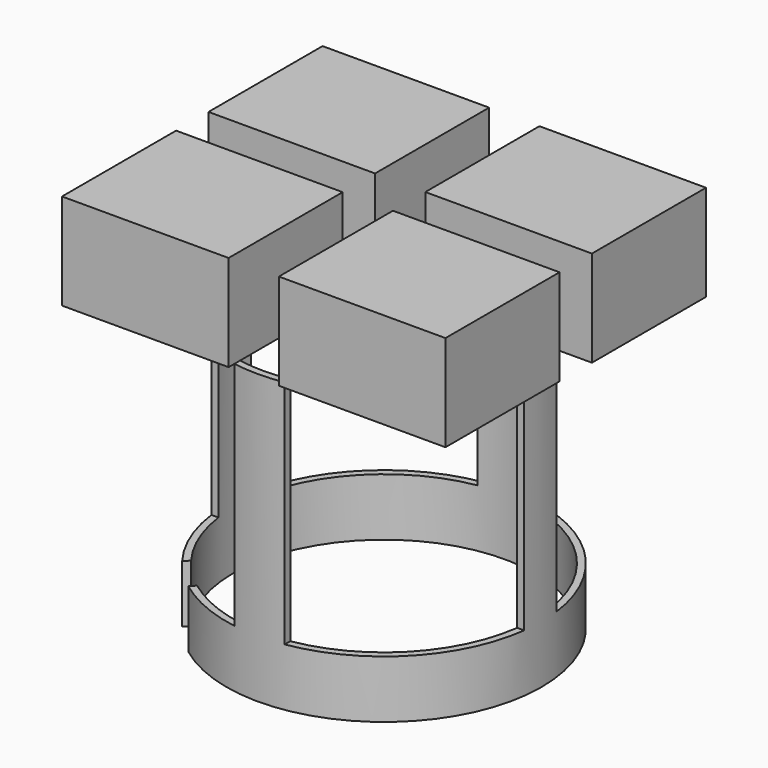
from build123d import *

# Parameters (mm, degrees)
F0_R      = 41
F1_DEPTH  = 75
F2_T      = -1.8
F3_W      = 43.3271373622
F3_H      = 37.0817845687
F4_DEPTH  = 25
F5_FACE_W = 43.3271373622
F5_FACE_H = 37.0817845687
F4_FACE_W = 43.3271373622
F4_FACE_H = 37.0817845687
F6_FACE_W = 43.3271373622
F6_FACE_H = 37.0817845687
F7_DEPTH  = 60
F10_DEPTH = 25


with BuildPart() as f1:
    # F0 (on Top) → F1 (new body)
    with BuildSketch(Plane.XY):
        Circle(F0_R)
    extrude(amount=F1_DEPTH)

    # F2
    f2_openings = [f1.faces().sort_by_distance(p)[0] for p in [
        (0, 0, 75),
        (0, 0, 0),
    ]]
    offset(amount=F2_T, openings=f2_openings)

    # F5_face (on face) + F4_face (on face) + F6_face (on face) → F7 (cut)
    with BuildSketch(Plane(origin=(28.2016734127, 23.8104094751, 75), x_dir=(1, 0, 0), z_dir=(0, 0, -1))):
        Rectangle(F5_FACE_W, F5_FACE_H)
    with BuildSketch(Plane(origin=(-28.2016734127, 23.8104094751, 75), x_dir=(1, 0, 0), z_dir=(0, 0, -1))):
        Rectangle(F4_FACE_W, F4_FACE_H)
    with BuildSketch(Plane(origin=(-28.2016734127, -23.8104094751, 75), x_dir=(1, 0, 0), z_dir=(0, 0, -1))):
        Rectangle(F6_FACE_W, F6_FACE_H)
        with Locations((56.4033468254, 0)):
            Rectangle(F6_FACE_W, F6_FACE_H)
    extrude(amount=F7_DEPTH, mode=Mode.SUBTRACT)

    # F9 (on face) → F10 (cut)
    with BuildSketch(Plane(origin=(0, 0, 0), x_dir=(1, 0, 0), z_dir=(0, 0, -1))):
        with BuildLine():
            Line((-26.0766707361, 33.9554976672), (-29.992537573, 30.0396308303))
            Line((-29.992537573, 30.0396308303), (-27.9037735724, 30.0396308303))
            ThreePointArc((-27.9037735724, 30.0396308303), (-26.3760293541, 31.3895695337), (-24.7830693928, 32.6618963239))
            Line((-24.7830693928, 32.6618963239), (-26.0766707361, 33.9554976672))
        make_face()
        with BuildLine():
            ThreePointArc((-24.7830693928, 32.6618963239), (-26.3760293541, 31.3895695337), (-27.9037735724, 30.0396308303))
            Line((-27.9037735724, 30.0396308303), (-25.184530561, 30.0396308303))
            ThreePointArc((-25.184530561, 30.0396308303), (-24.3503464301, 30.7197107528), (-23.497806174, 31.3766331051))
            Line((-23.497806174, 31.3766331051), (-24.7830693928, 32.6618963239))
        make_face()
        with BuildLine():
            Line((-25.184530561, 30.0396308303), (-27.9037735724, 30.0396308303))
            ThreePointArc((-27.9037735724, 30.0396308303), (-28.9669254959, 29.0158099545), (-29.992537573, 27.9543858801))
            Line((-29.992537573, 27.9543858801), (-29.992537573, 25.2405960693))
            ThreePointArc((-29.992537573, 25.2405960693), (-27.6926866813, 27.7444607872), (-25.184530561, 30.0396308303))
        make_face()
        with BuildLine():
            Line((-29.992537573, 25.2405960693), (-29.992537573, 27.9543858801))
            ThreePointArc((-29.992537573, 27.9543858801), (-31.3456683019, 26.4281872005), (-32.6212227873, 24.8365823708))
            Line((-32.6212227873, 24.8365823708), (-31.3362602205, 23.551619804))
            ThreePointArc((-31.3362602205, 23.551619804), (-30.6760251647, 24.4053576105), (-29.992537573, 25.2405960693))
        make_face()
    extrude(amount=-F10_DEPTH, mode=Mode.SUBTRACT)


with BuildPart() as f4:
    # F3 (on face) → F4 (new body)
    with BuildSketch(Plane.XY.offset(75)):
        with Locations((-28.2016734127, 23.8104094751)):
            Rectangle(F3_W, F3_H)
    extrude(amount=F4_DEPTH)


with BuildPart() as f5_1:
    # F5: instance of F4
    add(f4.part.mirror(Plane.YZ))


with BuildPart() as f6_1:
    # F6: instance of F4
    add(f4.part.mirror(Plane.XZ))


with BuildPart() as f6_2:
    # F6: instance of F5_1
    add(f5_1.part.mirror(Plane.XZ))


solid = Compound([f1.part, f4.part, f5_1.part, f6_1.part, f6_2.part])
